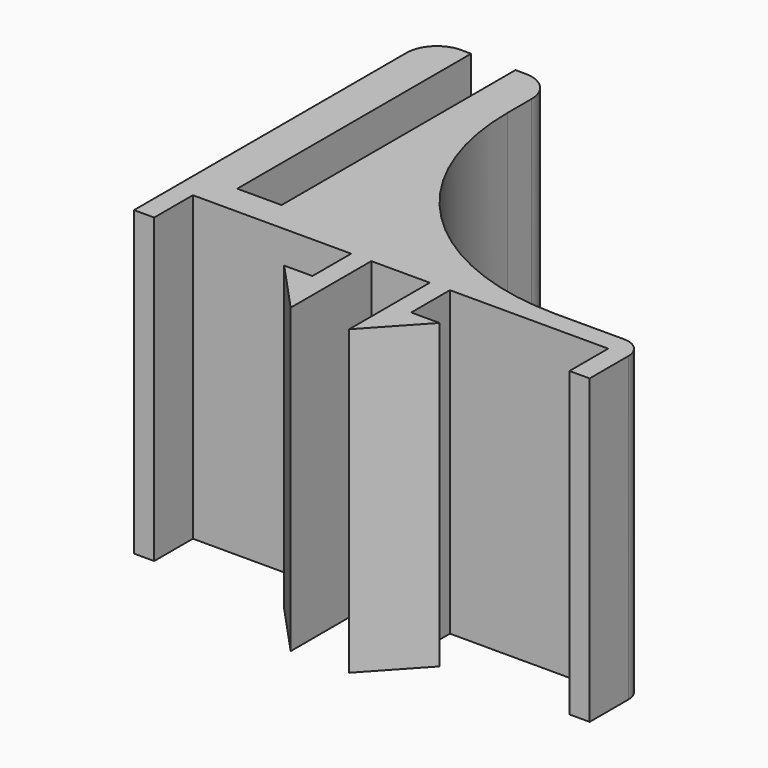
from build123d import *

# Parameters (mm, degrees)
F0_W     = 1
F0_H     = 2.4
F1_DEPTH = 15


# Not quite as in the source:
# - a feature names something its author has since deleted; it is built from what else it names


with BuildPart() as f1:
    # F0 (on Top) → F1 (new body)
    with BuildSketch(Plane.XY):
        with Locations((10.8, -6.7)):
            Rectangle(F0_W, F0_H)
        with Locations((-10.8, -6.7)):
            Rectangle(F0_W, F0_H)
        Polygon((-2.45, -8.5), (-2.45, -7.9), (-3.85, -7.9), (-1.45, -10.5), (-1.45, -8.5), align=None)
        with BuildLine():
            Line((10.3, -4.5), (10.3, -5.5))
            Line((10.3, -5.5), (11.3, -5.5))
            ThreePointArc((11.3, -5.5), (11.0071067812, -4.7928932188), (10.3, -4.5))
        make_face()
        Polygon((-1.45, -5.5), (-2.45, -5.5), (-2.45, -7.9), (-2.45, -8.5), (-1.45, -8.5), align=None)
        Polygon((2.45, -5.5), (1.45, -5.5), (1.45, -8.5), (2.45, -8.5), (2.45, -7.9), align=None)
        with BuildLine():
            Line((-11.3, -5.5), (-10.3, -5.5))
            Line((-10.3, -5.5), (-2.45, -5.5))
            Line((-2.45, -5.5), (-1.45, -5.5))
            Line((-1.45, -5.5), (1.45, -5.5))
            Line((1.45, -5.5), (2.45, -5.5))
            Line((2.45, -5.5), (10.3, -5.5))
            Line((10.3, -5.5), (10.3, -4.5))
            Line((10.3, -4.5), (6.9, -4.5))
            ThreePointArc((6.9, -4.5), (-1.5852813742, -0.9852813742), (-5.1, 7.5))
            Line((-5.1, 7.5), (-5.1, 9))
            ThreePointArc((-5.1, 9), (-5.5393398282, 10.0606601718), (-6.6, 10.5))
            Line((-6.6, 10.5), (-7.1, 10.5))
            Line((-7.1, 10.5), (-7.1, -4))
            Line((-7.1, -4), (-9.3, -4))
            Line((-9.3, -4), (-9.3, 10.5))
            Line((-9.3, 10.5), (-9.8, 10.5))
            ThreePointArc((-9.8, 10.5), (-10.8606601718, 10.0606601718), (-11.3, 9))
            Line((-11.3, 9), (-11.3, -5.5))
        make_face()
        Polygon((2.45, -8.5), (1.45, -8.5), (1.45, -10.5), (3.85, -7.9), (2.45, -7.9), align=None)
    extrude(amount=F1_DEPTH)


solid = f1.part
